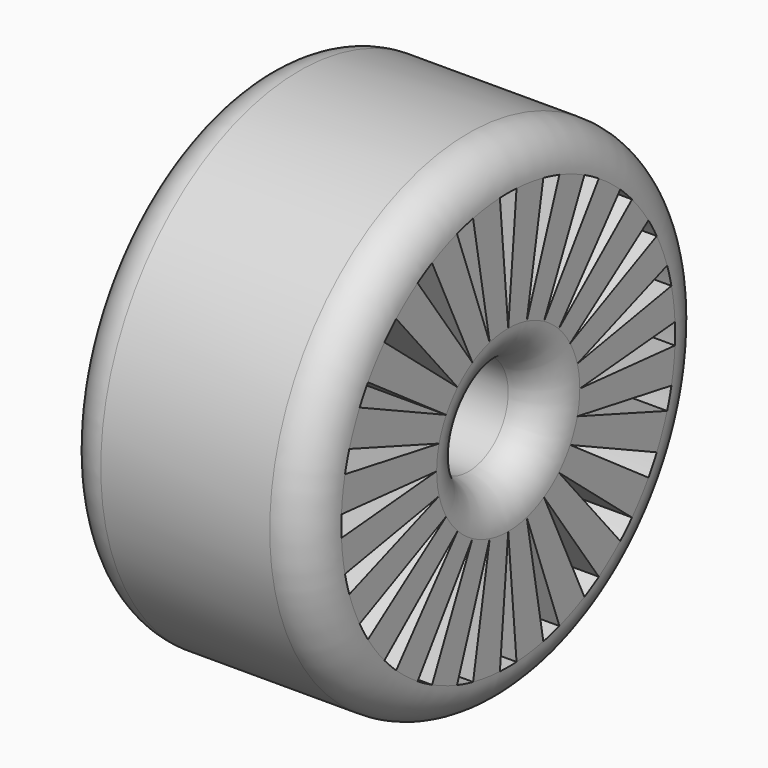
from build123d import *

# Parameters (mm, degrees)
F0_R            = 10
F0_R_2          = 5
F1_DEPTH        = 12.5
F0_R_3          = 25
F2_DEPTH        = 12.5
F3_R            = 5
F4_R            = 4
F6_DEPTH        = 25.001
F6_COPIES_COUNT = 24


# Not quite as in the source:
# - a pattern or mirror of a feature is missing from the dataset's text; its kind, count and spacing are read off the source's solid


with BuildPart() as f1:
    # F0 (on Right) → F1 (new body, symmetric)
    with BuildSketch(Plane.YZ):
        Circle(F0_R)
        Circle(F0_R_2, mode=Mode.SUBTRACT)
    extrude(amount=F1_DEPTH, both=True)

    # F0 (on Right) → F2 (join, symmetric)
    with BuildSketch(Plane.YZ):
        Circle(F0_R_3)
        Circle(F0_R, mode=Mode.SUBTRACT)
    extrude(amount=F2_DEPTH, both=True)

    # F3
    f3_edges = [f1.edges().sort_by_distance(p)[0] for p in [
        (-12.5, -5, 0),
    ]]
    fillet(f3_edges, radius=F3_R)

    # F4
    f4_edges = [f1.edges().sort_by_distance(p)[0] for p in [
        (12.5, -25, 0),
        (-12.5, -25, 0),
        (12.5, -5, 0),
    ]]
    fillet(f4_edges, radius=F4_R)

    # F5 (on face) → F6 (cut, through all)
    with BuildSketch(Plane.YZ.offset(12.5)):
        with BuildLine():
            Line((-1.04757655, 20.9738547571), (0, 9))
            Line((0, 9), (1.04757655, 20.9738547571))
            ThreePointArc((1.04757655, 20.9738547571), (0, 21), (-1.04757655, 20.9738547571))
        make_face()
    f6 = extrude(amount=-F6_DEPTH, mode=Mode.SUBTRACT)

    # F6_copies: F6 ×24 about axis
    f6_copies_axis = Axis((0, 0, 0), (1, 0, 0))
    for i in range(1, F6_COPIES_COUNT):
        add(f6.rotate(f6_copies_axis, i * 360 / F6_COPIES_COUNT), mode=Mode.SUBTRACT)


solid = f1.part
